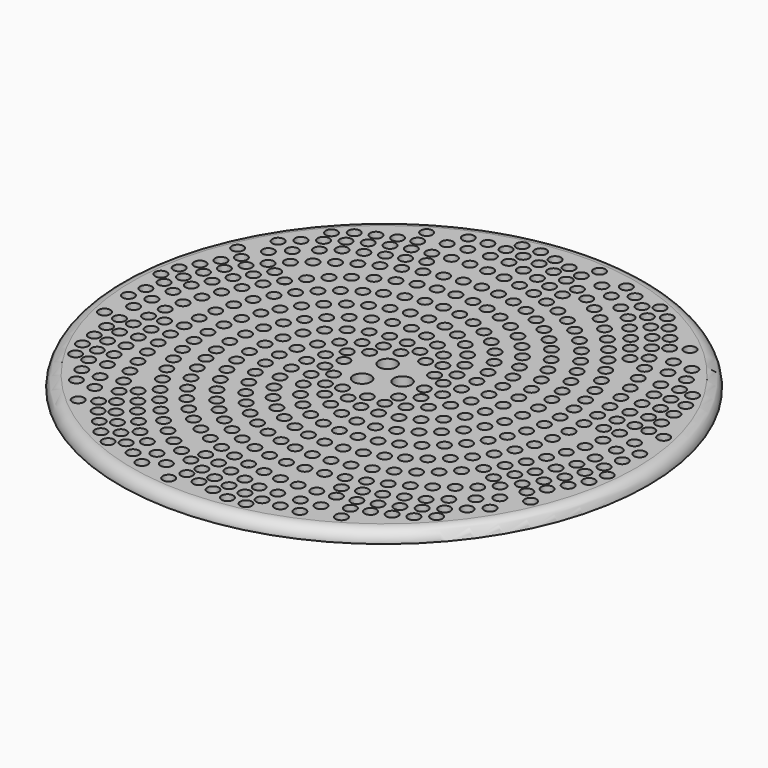
from build123d import *

# Parameters (mm, degrees)
F0_R      = 45
F1_DEPTH  = 2
F2_R      = 5.25
F3_DEPTH  = 1
F4_R      = 3.75
F5_DEPTH  = 5
F6_R      = 2
F7_R      = 1.99999
F8_R      = 1
F9_DEPTH  = 25
F10_R     = 1
F10_R_2   = 1.5
F11_DEPTH = 25


# Not quite as in the source:
# - a fillet or chamfer is up to 0.001 mm smaller than in the source, because OpenCascade refuses the exact size


with BuildPart() as f1:
    # F0 (on Top) → F1 (new body)
    with BuildSketch(Plane.XY):
        Circle(F0_R)
    extrude(amount=F1_DEPTH)

    # F2 (on face) → F3 (cut)
    with BuildSketch(Plane(origin=(0, 0, 0), x_dir=(1, 0, 0), z_dir=(0, 0, -1))):
        with Locations((0, 35)):
            Circle(F2_R)
        with Locations((-30.3108891325, -17.5)):
            Circle(F2_R)
        with Locations((30.3108891325, -17.5)):
            Circle(F2_R)
    extrude(amount=-F3_DEPTH, mode=Mode.SUBTRACT)

    # F4 (on face) → F5 (join)
    with BuildSketch(Plane(origin=(0, 0, 1), x_dir=(1, 0, 0), z_dir=(0, 0, -1))):
        with Locations((0, 35)):
            Circle(F4_R)
        with Locations((30.3108891325, -17.5)):
            Circle(F4_R)
        with Locations((-30.3108891325, -17.5)):
            Circle(F4_R)
    extrude(amount=F5_DEPTH)

    # F6
    f6_edges = [f1.edges().sort_by_distance(p)[0] for p in [
        (-34.060889, 17.5, -4),
        (-3.75, -35, -4),
        (26.560889, 17.5, -4),
    ]]
    fillet(f6_edges, radius=F6_R)

    # F7 (radius 2 in the source; OpenCascade refuses exactly that, so slightly less here)
    f7_edges = [f1.edges().sort_by_distance(p)[0] for p in [
        (-45, 0, 2),
    ]]
    fillet(f7_edges, radius=F7_R)

    # F8 (on face) → F9 (cut)
    with BuildSketch(Plane.XY.offset(2)):
        with Locations((-40.8493989427, -3.4236625268)):
            Circle(F8_R)
        with Locations((-37.2194312295, 8.0217761925)):
            Circle(F8_R)
        with Locations((-39.4834812949, 2.4710397464)):
            Circle(F8_R)
        with Locations((-38.4680309655, 5.2939567888)):
            Circle(F8_R)
        with Locations((-40.2713256638, -0.4236625268)):
            Circle(F8_R)
        with Locations((-35.7373339506, 10.6301066271)):
            Circle(F8_R)
        with Locations((-34.027593705, 13.0952208826)):
            Circle(F8_R)
        with Locations((-32.1025009246, 15.3960941487)):
            Circle(F8_R)
        with Locations((-22.7184350173, 22.804778367)):
            Circle(F8_R)
        with Locations((-27.6942880126, 19.4590303855)):
            Circle(F8_R)
        with Locations((-25.2667541466, 21.2217213197)):
            Circle(F8_R)
        with Locations((-29.981542035, 17.5177758847)):
            Circle(F8_R)
        with Locations((-20.0643504801, 24.2032901724)):
            Circle(F8_R)
        with Locations((-17.3167057976, 25.4076359278)):
            Circle(F8_R)
        with Locations((-14.4864313326, 26.4023954226)):
            Circle(F8_R)
        with Locations((-11.5849426999, 27.1648675298)):
            Circle(F8_R)
        with Locations((-8.626607772, 27.6631189269)):
            Circle(F8_R)
        with Locations((-5.6326711003, 27.8537578673)):
            Circle(F8_R)
        with Locations((5.9110662235, 25.0201439515)):
            Circle(F8_R)
        with Locations((0.3145207901, 27.1521286585)):
            Circle(F8_R)
        with Locations((3.177785049, 26.256741712)):
            Circle(F8_R)
        with Locations((-2.6372636774, 27.6878230277)):
            Circle(F8_R)
        with Locations((8.4765099907, 23.4649917798)):
            Circle(F8_R)
        with Locations((10.8377438023, 21.6144310845)):
            Circle(F8_R)
        with Locations((12.8210696775, 19.6416883073)):
            Circle(F8_R)
        with Locations((14.6696584192, 17.2789103524)):
            Circle(F8_R)
        with Locations((16.1762201169, 14.6846336033)):
            Circle(F8_R)
        with Locations((17.2872605499, 11.8979529334)):
            Circle(F8_R)
        with Locations((17.1563704418, 0.1090617956)):
            Circle(F8_R)
        with Locations((18.1599637889, 6.0055567892)):
            Circle(F8_R)
        with Locations((17.8915320419, 3.0175901902)):
            Circle(F8_R)
        with Locations((17.9579806895, 8.973891632)):
            Circle(F8_R)
        with Locations((15.9391579938, -2.6329071787)):
            Circle(F8_R)
        with Locations((14.2051991524, -5.0810466225)):
            Circle(F8_R)
        with Locations((6.3437518281, -9.104549132)):
            Circle(F8_R)
        with Locations((3.343753197, -9.1074149941)):
            Circle(F8_R)
        with Locations((9.2585771237, -8.3947650127)):
            Circle(F8_R)
        with Locations((11.9383022455, -7.0460347685)):
            Circle(F8_R)
        with Locations((0.4738705573, -8.2334735575)):
            Circle(F8_R)
        with Locations((-1.9367000752, -6.4476546346)):
            Circle(F8_R)
        with Locations((13.7998447247, 1.3167961267)):
            Circle(F8_R)
        with Locations((-9.9243185953, 23.71615921)):
            Circle(F8_R)
        with Locations((10.4837227456, -3.6369712052)):
            Circle(F8_R)
        with Locations((6.9922463043, 19.7868429251)):
            Circle(F8_R)
        with Locations((9.2535904055, 17.8154670462)):
            Circle(F8_R)
        with Locations((-25.3395240375, 15.1673810139)):
            Circle(F8_R)
        with Locations((-34.5522673419, -3.4505298548)):
            Circle(F8_R)
        with Locations((-30.4587375398, 7.7873437602)):
            Circle(F8_R)
        with Locations((4.455425912, 21.3882617638)):
            Circle(F8_R)
        with Locations((-28.9437429708, 10.3767049663)):
            Circle(F8_R)
        with Locations((-31.0354796126, -26.7804754307)):
            Circle(F8_R)
        with Locations((-34.8262341288, -15.3872795106)):
            Circle(F8_R)
        with Locations((-33.3952480854, -21.2086948657)):
            Circle(F8_R)
        with Locations((-32.3311642628, -24.0136414995)):
            Circle(F8_R)
        with Locations((13.8156903342, 10.1724943747)):
            Circle(F8_R)
        with Locations((-35.1603304054, -12.4059409391)):
            Circle(F8_R)
        with Locations((-35.2260792953, -9.4066615117)):
            Circle(F8_R)
        with Locations((-35.0210658934, -6.4136747919)):
            Circle(F8_R)
        with Locations((-31.7839124205, 5.0958921935)):
            Circle(F8_R)
        with Locations((-3.9367249114, 23.8567080462)):
            Circle(F8_R)
        with Locations((-33.8428807338, -0.5356077906)):
            Circle(F8_R)
        with Locations((-32.9150483173, 2.3173077369)):
            Circle(F8_R)
        with Locations((2.2230130322, -6.3546259156)):
            Circle(F8_R)
        with Locations((12.4246653077, -1.3494524685)):
            Circle(F8_R)
        with Locations((-27.2387077905, 12.8450758935)):
            Circle(F8_R)
        with Locations((-6.9347354779, 23.9659446861)):
            Circle(F8_R)
        with Locations((-18.4080851774, 20.8497746707)):
            Circle(F8_R)
        with Locations((14.4426337033, 7.2387353505)):
            Circle(F8_R)
        with Locations((14.4788117937, 4.2389535008)):
            Circle(F8_R)
        with Locations((12.7008584661, 12.957660421)):
            Circle(F8_R)
        with Locations((1.711714282, 22.6015409944)):
            Circle(F8_R)
        with Locations((-34.233000518, -18.3280402766)):
            Circle(F8_R)
        with Locations((8.0583573814, -5.4026446886)):
            Circle(F8_R)
        with Locations((-15.7051681295, 22.1514042001)):
            Circle(F8_R)
        with Locations((-1.172631462, 23.4264953138)):
            Circle(F8_R)
        with Locations((11.1617416099, 15.5327564005)):
            Circle(F8_R)
        with Locations((-23.239045629, 17.3093405036)):
            Circle(F8_R)
        with Locations((-12.8624434425, 23.1100054487)):
            Circle(F8_R)
        with Locations((5.2228836663, -6.3824859057)):
            Circle(F8_R)
        with Locations((-20.9289547392, 19.2233624681)):
            Circle(F8_R)
        with Locations((10.3903155584, 9.1766556577)):
            Circle(F8_R)
        with Locations((-21.9689510258, 13.3534077328)):
            Circle(F8_R)
        with Locations((10.619267903, 3.219806106)):
            Circle(F8_R)
        with Locations((-5.9735683718, 20.1178314495)):
            Circle(F8_R)
        with Locations((-2.9853568954, 19.8521395742)):
            Circle(F8_R)
        with Locations((-29.4152684516, -2.623529529)):
            Circle(F8_R)
        with Locations((-25.9252009125, -23.100850469)):
            Circle(F8_R)
        with Locations((-29.2189221137, -11.6031032863)):
            Circle(F8_R)
        with Locations((-8.967189557, 19.9223008908)):
            Circle(F8_R)
        with Locations((-29.5152540908, -8.617774601)):
            Circle(F8_R)
        with Locations((-9.3670619276, -39.908056955)):
            Circle(F8_R)
        with Locations((-19.1305992911, -32.9189174351)):
            Circle(F8_R)
        with Locations((-14.55116517, -36.7874288961)):
            Circle(F8_R)
        with Locations((-12.0415970093, -38.431225613)):
            Circle(F8_R)
        with Locations((5.1978860969, 16.350379853)):
            Circle(F8_R)
        with Locations((-21.153275701, -30.7033407289)):
            Circle(F8_R)
        with Locations((-22.9693998852, -28.3155189292)):
            Circle(F8_R)
        with Locations((-24.5627740133, -25.7736379547)):
            Circle(F8_R)
        with Locations((-28.7090155745, -14.5594515948)):
            Circle(F8_R)
        with Locations((-17.2074985133, 16.9865333939)):
            Circle(F8_R)
        with Locations((-27.0646432919, -20.3256619954)):
            Circle(F8_R)
        with Locations((-27.9909127721, -17.4722386391)):
            Circle(F8_R)
        with Locations((5.5336107188, -3.8343460826)):
            Circle(F8_R)
        with Locations((10.844953643, 6.2113050524)):
            Circle(F8_R)
        with Locations((-29.5867236821, -5.6186260389)):
            Circle(F8_R)
        with Locations((-19.6971476969, 15.3127212949)):
            Circle(F8_R)
        with Locations((-27.1476438075, 6.0478210472)):
            Circle(F8_R)
        with Locations((7.4295142253, 14.3454270114)):
            Circle(F8_R)
        with Locations((9.2220104465, 11.9398174636)):
            Circle(F8_R)
        with Locations((2.6588886425, 17.9483447858)):
            Circle(F8_R)
        with Locations((-11.900046532, 19.2911511746)):
            Circle(F8_R)
        with Locations((-16.9221274095, -34.9493489036)):
            Circle(F8_R)
        with Locations((9.6949429396, 0.3657522589)):
            Circle(F8_R)
        with Locations((-25.7260166227, 8.6895962359)):
            Circle(F8_R)
        with Locations((-14.7184272393, 18.2631773478)):
            Circle(F8_R)
        with Locations((-0.0998864904, 19.1269710057)):
            Circle(F8_R)
        with Locations((-28.9749579218, 0.3439823307)):
            Circle(F8_R)
        with Locations((-23.9896557173, 11.1360325842)):
            Circle(F8_R)
        with Locations((7.976932734, -2.0936055706)):
            Circle(F8_R)
        with Locations((-28.2310890167, 3.2502959841)):
            Circle(F8_R)
        with Locations((3.0120390027, 13.5313446305)):
            Circle(F8_R)
        with Locations((-25.6221908617, -2.1098916326)):
            Circle(F8_R)
        with Locations((6.698613657, 8.8467269218)):
            Circle(F8_R)
        with Locations((-16.6576829639, 12.7644921402)):
            Circle(F8_R)
        with Locations((-14.0839993308, 14.3059695343)):
            Circle(F8_R)
        with Locations((-22.2553801054, -19.4123409623)):
            Circle(F8_R)
        with Locations((-7.3955888997, -33.927431373)):
            Circle(F8_R)
        with Locations((-16.8184715547, -26.5615592524)):
            Circle(F8_R)
        with Locations((-18.9646433987, 10.8466982116)):
            Circle(F8_R)
        with Locations((-18.8129413347, -24.3205571782)):
            Circle(F8_R)
        with Locations((15.879255039, -37.7921171474)):
            Circle(F8_R)
        with Locations((3.8722742507, -37.8766477722)):
            Circle(F8_R)
        with Locations((9.8509682644, -38.3146154469)):
            Circle(F8_R)
        with Locations((12.847451023, -38.1693877717)):
            Circle(F8_R)
        with Locations((-5.4053339597, 16.2829759564)):
            Circle(F8_R)
        with Locations((0.9336113478, -37.2731079285)):
            Circle(F8_R)
        with Locations((-1.9391904202, -36.4088105248)):
            Circle(F8_R)
        with Locations((-4.722337318, -35.2889474326)):
            Circle(F8_R)
        with Locations((-14.6682505627, -28.6535797316)):
            Circle(F8_R)
        with Locations((-23.9055925445, 3.6280803362)):
            Circle(F8_R)
        with Locations((-9.9486320059, -32.3520041617)):
            Circle(F8_R)
        with Locations((-12.3751999241, -30.5879837145)):
            Circle(F8_R)
        with Locations((6.7305571913, 0.1505236293)):
            Circle(F8_R)
        with Locations((5.1228382931, 11.3995551578)):
            Circle(F8_R)
        with Locations((-20.6336167429, -21.9362037945)):
            Circle(F8_R)
        with Locations((-24.9359189771, 0.8105588293)):
            Circle(F8_R)
        with Locations((-25.5177252176, -11.0641946584)):
            Circle(F8_R)
        with Locations((-2.421427167, 15.9726531371)):
            Circle(F8_R)
        with Locations((0.4427145534, 15.0800769747)):
            Circle(F8_R)
        with Locations((-8.3986862702, 16.0833714841)):
            Circle(F8_R)
        with Locations((-20.9663940384, 8.6121972882)):
            Circle(F8_R)
        with Locations((6.8524232075, -38.2211941341)):
            Circle(F8_R)
        with Locations((7.6283898139, 5.9944442749)):
            Circle(F8_R)
        with Locations((-25.9204011611, -8.091342142)):
            Circle(F8_R)
        with Locations((-22.6422840721, 6.1239463775)):
            Circle(F8_R)
        with Locations((-11.3233613464, 15.4153327886)):
            Circle(F8_R)
        with Locations((-23.6434211111, -16.7527654009)):
            Circle(F8_R)
        with Locations((-25.9536348865, -5.0915262277)):
            Circle(F8_R)
        with Locations((7.6840646233, 2.9949609334)):
            Circle(F8_R)
        with Locations((-24.7499068293, -13.9642730923)):
            Circle(F8_R)
        with Locations((-5.5167340766, 12.717519868)):
            Circle(F8_R)
        with Locations((-19.4886246546, -16.767284107)):
            Circle(F8_R)
        with Locations((0.2193166715, 11.0944987427)):
            Circle(F8_R)
        with Locations((-20.9791288377, 0.5355506824)):
            Circle(F8_R)
        with Locations((-19.8030327194, 3.2954053743)):
            Circle(F8_R)
        with Locations((-6.5946929914, -28.7862979492)):
            Circle(F8_R)
        with Locations((13.9588867059, -31.7948866435)):
            Circle(F8_R)
        with Locations((2.0060634993, -31.3744023783)):
            Circle(F8_R)
        with Locations((-21.7182480467, -2.3719745187)):
            Circle(F8_R)
        with Locations((-0.9247244171, -30.7337135386)):
            Circle(F8_R)
        with Locations((35.0602362968, -21.2408730963)):
            Circle(F8_R)
        with Locations((25.3960706425, -28.3667860402)):
            Circle(F8_R)
        with Locations((30.4903666439, -25.2069211629)):
            Circle(F8_R)
        with Locations((32.8292094332, -23.3281411313)):
            Circle(F8_R)
        with Locations((-13.9439001643, 9.9960286825)):
            Circle(F8_R)
        with Locations((22.663890594, -29.6058147657)):
            Circle(F8_R)
        with Locations((19.8317238747, -30.5951739899)):
            Circle(F8_R)
        with Locations((16.9218717264, -31.3250784185)):
            Circle(F8_R)
        with Locations((4.9752876087, -31.8030143102)):
            Circle(F8_R)
        with Locations((-21.4725627448, -11.116176096)):
            Circle(F8_R)
        with Locations((10.9674185648, -32.0209803425)):
            Circle(F8_R)
        with Locations((7.9674186773, -32.0201586583)):
            Circle(F8_R)
        with Locations((5.35665958, 4.0778984309)):
            Circle(F8_R)
        with Locations((-2.5560271659, 12.2335626496)):
            Circle(F8_R)
        with Locations((-3.7991695187, -29.8748972847)):
            Circle(F8_R)
        with Locations((-20.6500167488, -14.0012095593)):
            Circle(F8_R)
        with Locations((-14.1409029101, -23.9500640627)):
            Circle(F8_R)
        with Locations((-11.3474656827, 11.4988686549)):
            Circle(F8_R)
        with Locations((-8.5056832518, 12.4602596345)):
            Circle(F8_R)
        with Locations((-16.2482484885, 8.0750969292)):
            Circle(F8_R)
        with Locations((-22.0242916437, -5.3563232444)):
            Circle(F8_R)
        with Locations((28.0095810645, -26.8938422959)):
            Circle(F8_R)
        with Locations((2.6480510587, 9.3334623216)):
            Circle(F8_R)
        with Locations((-16.2140734581, -21.7816628362)):
            Circle(F8_R)
        with Locations((-21.9175579723, -8.3544239638)):
            Circle(F8_R)
        with Locations((-18.221697035, 5.8155613941)):
            Circle(F8_R)
        with Locations((-9.2809010463, -27.450526155)):
            Circle(F8_R)
        with Locations((-18.0042076607, -19.3742950752)):
            Circle(F8_R)
        with Locations((4.4561449982, 6.9395541559)):
            Circle(F8_R)
        with Locations((-11.8151014515, -25.8449644756)):
            Circle(F8_R)
        with Locations((-11.9383022455, 7.0460347685)):
            Circle(F8_R)
        with Locations((-5.9110662235, -25.0201439515)):
            Circle(F8_R)
        with Locations((-6.3437518281, 9.104549132)):
            Circle(F8_R)
        with Locations((-17.2872605499, -11.8979529334)):
            Circle(F8_R)
        with Locations((-17.9579806895, -8.973891632)):
            Circle(F8_R)
        with Locations((11.5849426999, -27.1648675298)):
            Circle(F8_R)
        with Locations((29.981542035, -17.5177758847)):
            Circle(F8_R)
        with Locations((20.0643504801, -24.2032901724)):
            Circle(F8_R)
        with Locations((-16.1762201169, -14.6846336033)):
            Circle(F8_R)
        with Locations((17.3167057976, -25.4076359278)):
            Circle(F8_R)
        with Locations((40.8493989427, 3.4236625268)):
            Circle(F8_R)
        with Locations((37.2194312295, -8.0217761925)):
            Circle(F8_R)
        with Locations((39.4834812949, -2.4710397464)):
            Circle(F8_R)
        with Locations((40.2713256638, 0.4236625268)):
            Circle(F8_R)
        with Locations((-17.1563704418, -0.1090617956)):
            Circle(F8_R)
        with Locations((35.7373339506, -10.6301066271)):
            Circle(F8_R)
        with Locations((34.027593705, -13.0952208826)):
            Circle(F8_R)
        with Locations((32.1025009246, -15.3960941487)):
            Circle(F8_R)
        with Locations((22.7184350173, -22.804778367)):
            Circle(F8_R)
        with Locations((-10.8377438023, -21.6144310845)):
            Circle(F8_R)
        with Locations((27.6942880126, -19.4590303855)):
            Circle(F8_R)
        with Locations((25.2667541466, -21.2217213197)):
            Circle(F8_R)
        with Locations((1.9367000752, 6.4476546346)):
            Circle(F8_R)
        with Locations((-9.2585771237, 8.3947650127)):
            Circle(F8_R)
        with Locations((14.4864313326, -26.4023954226)):
            Circle(F8_R)
        with Locations((-8.4765099907, -23.4649917798)):
            Circle(F8_R)
        with Locations((2.6372636774, -27.6878230277)):
            Circle(F8_R)
        with Locations((-15.9391579938, 2.6329071787)):
            Circle(F8_R)
        with Locations((-14.2051991524, 5.0810466225)):
            Circle(F8_R)
        with Locations((-17.8915320419, -3.0175901902)):
            Circle(F8_R)
        with Locations((-14.6696584192, -17.2789103524)):
            Circle(F8_R)
        with Locations((38.4680309655, -5.2939567888)):
            Circle(F8_R)
        with Locations((-3.343753197, 9.1074149941)):
            Circle(F8_R)
        with Locations((-0.3145207901, -27.1521286585)):
            Circle(F8_R)
        with Locations((-12.8210696775, -19.6416883073)):
            Circle(F8_R)
        with Locations((-18.1599637889, -6.0055567892)):
            Circle(F8_R)
        with Locations((8.626607772, -27.6631189269)):
            Circle(F8_R)
        with Locations((-3.177785049, -26.256741712)):
            Circle(F8_R)
        with Locations((-0.4738705573, 8.2334735575)):
            Circle(F8_R)
        with Locations((5.6326711003, -27.8537578673)):
            Circle(F8_R)
        with Locations((-13.7998447247, -1.3167961267)):
            Circle(F8_R)
        with Locations((9.9243185953, -23.71615921)):
            Circle(F8_R)
        with Locations((-10.4837227456, 3.6369712052)):
            Circle(F8_R)
        with Locations((-6.9922463043, -19.7868429251)):
            Circle(F8_R)
        with Locations((-9.2535904055, -17.8154670462)):
            Circle(F8_R)
        with Locations((25.3395240375, -15.1673810139)):
            Circle(F8_R)
        with Locations((34.5522673419, 3.4505298548)):
            Circle(F8_R)
        with Locations((30.4587375398, -7.7873437602)):
            Circle(F8_R)
        with Locations((-4.455425912, -21.3882617638)):
            Circle(F8_R)
        with Locations((28.9437429708, -10.3767049663)):
            Circle(F8_R)
        with Locations((31.0354796126, 26.7804754307)):
            Circle(F8_R)
        with Locations((34.8262341288, 15.3872795106)):
            Circle(F8_R)
        with Locations((33.3952480854, 21.2086948657)):
            Circle(F8_R)
        with Locations((32.3311642628, 24.0136414995)):
            Circle(F8_R)
        with Locations((-13.8156903342, -10.1724943747)):
            Circle(F8_R)
        with Locations((35.1603304054, 12.4059409391)):
            Circle(F8_R)
        with Locations((35.2260792953, 9.4066615117)):
            Circle(F8_R)
        with Locations((35.0210658934, 6.4136747919)):
            Circle(F8_R)
        with Locations((31.7839124205, -5.0958921935)):
            Circle(F8_R)
        with Locations((3.9367249114, -23.8567080462)):
            Circle(F8_R)
        with Locations((33.8428807338, 0.5356077906)):
            Circle(F8_R)
        with Locations((32.9150483173, -2.3173077369)):
            Circle(F8_R)
        with Locations((-2.2230130322, 6.3546259156)):
            Circle(F8_R)
        with Locations((-12.4246653077, 1.3494524685)):
            Circle(F8_R)
        with Locations((27.2387077905, -12.8450758935)):
            Circle(F8_R)
        with Locations((6.9347354779, -23.9659446861)):
            Circle(F8_R)
        with Locations((18.4080851774, -20.8497746707)):
            Circle(F8_R)
        with Locations((-14.4426337033, -7.2387353505)):
            Circle(F8_R)
        with Locations((-14.4788117937, -4.2389535008)):
            Circle(F8_R)
        with Locations((-12.7008584661, -12.957660421)):
            Circle(F8_R)
        with Locations((-1.711714282, -22.6015409944)):
            Circle(F8_R)
        with Locations((34.233000518, 18.3280402766)):
            Circle(F8_R)
        with Locations((-8.0583573814, 5.4026446886)):
            Circle(F8_R)
        with Locations((15.7051681295, -22.1514042001)):
            Circle(F8_R)
        with Locations((1.172631462, -23.4264953138)):
            Circle(F8_R)
        with Locations((-11.1617416099, -15.5327564005)):
            Circle(F8_R)
        with Locations((23.239045629, -17.3093405036)):
            Circle(F8_R)
        with Locations((12.8624434425, -23.1100054487)):
            Circle(F8_R)
        with Locations((-5.2228836663, 6.3824859057)):
            Circle(F8_R)
        with Locations((20.9289547392, -19.2233624681)):
            Circle(F8_R)
        with Locations((-10.3903155584, -9.1766556577)):
            Circle(F8_R)
        with Locations((21.9689510258, -13.3534077328)):
            Circle(F8_R)
        with Locations((-10.619267903, -3.219806106)):
            Circle(F8_R)
        with Locations((5.9735683718, -20.1178314495)):
            Circle(F8_R)
        with Locations((2.9853568954, -19.8521395742)):
            Circle(F8_R)
        with Locations((29.4152684516, 2.623529529)):
            Circle(F8_R)
        with Locations((25.9252009125, 23.100850469)):
            Circle(F8_R)
        with Locations((29.2189221137, 11.6031032863)):
            Circle(F8_R)
        with Locations((8.967189557, -19.9223008908)):
            Circle(F8_R)
        with Locations((29.5152540908, 8.617774601)):
            Circle(F8_R)
        with Locations((9.3670619276, 39.908056955)):
            Circle(F8_R)
        with Locations((19.1305992911, 32.9189174351)):
            Circle(F8_R)
        with Locations((14.55116517, 36.7874288961)):
            Circle(F8_R)
        with Locations((12.0415970093, 38.431225613)):
            Circle(F8_R)
        with Locations((-5.1978860969, -16.350379853)):
            Circle(F8_R)
        with Locations((21.153275701, 30.7033407289)):
            Circle(F8_R)
        with Locations((22.9693998852, 28.3155189292)):
            Circle(F8_R)
        with Locations((24.5627740133, 25.7736379547)):
            Circle(F8_R)
        with Locations((28.7090155745, 14.5594515948)):
            Circle(F8_R)
        with Locations((17.2074985133, -16.9865333939)):
            Circle(F8_R)
        with Locations((27.0646432919, 20.3256619954)):
            Circle(F8_R)
        with Locations((27.9909127721, 17.4722386391)):
            Circle(F8_R)
        with Locations((-5.5336107188, 3.8343460826)):
            Circle(F8_R)
        with Locations((-10.844953643, -6.2113050524)):
            Circle(F8_R)
        with Locations((29.5867236821, 5.6186260389)):
            Circle(F8_R)
        with Locations((19.6971476969, -15.3127212949)):
            Circle(F8_R)
        with Locations((27.1476438075, -6.0478210472)):
            Circle(F8_R)
        with Locations((-7.4295142253, -14.3454270114)):
            Circle(F8_R)
        with Locations((-9.2220104465, -11.9398174636)):
            Circle(F8_R)
        with Locations((-2.6588886425, -17.9483447858)):
            Circle(F8_R)
        with Locations((11.900046532, -19.2911511746)):
            Circle(F8_R)
        with Locations((16.9221274095, 34.9493489036)):
            Circle(F8_R)
        with Locations((-9.6949429396, -0.3657522589)):
            Circle(F8_R)
        with Locations((25.7260166227, -8.6895962359)):
            Circle(F8_R)
        with Locations((14.7184272393, -18.2631773478)):
            Circle(F8_R)
        with Locations((0.0998864904, -19.1269710057)):
            Circle(F8_R)
        with Locations((28.9749579218, -0.3439823307)):
            Circle(F8_R)
        with Locations((23.9896557173, -11.1360325842)):
            Circle(F8_R)
        with Locations((-7.976932734, 2.0936055706)):
            Circle(F8_R)
        with Locations((28.2310890167, -3.2502959841)):
            Circle(F8_R)
        with Locations((-3.0120390027, -13.5313446305)):
            Circle(F8_R)
        with Locations((25.6221908617, 2.1098916326)):
            Circle(F8_R)
        with Locations((-6.698613657, -8.8467269218)):
            Circle(F8_R)
        with Locations((16.6576829639, -12.7644921402)):
            Circle(F8_R)
        with Locations((14.0839993308, -14.3059695343)):
            Circle(F8_R)
        with Locations((22.2553801054, 19.4123409623)):
            Circle(F8_R)
        with Locations((7.3955888997, 33.927431373)):
            Circle(F8_R)
        with Locations((16.8184715547, 26.5615592524)):
            Circle(F8_R)
        with Locations((18.9646433987, -10.8466982116)):
            Circle(F8_R)
        with Locations((18.8129413347, 24.3205571782)):
            Circle(F8_R)
        with Locations((-15.879255039, 37.7921171474)):
            Circle(F8_R)
        with Locations((-3.8722742507, 37.8766477722)):
            Circle(F8_R)
        with Locations((-9.8509682644, 38.3146154469)):
            Circle(F8_R)
        with Locations((-12.847451023, 38.1693877717)):
            Circle(F8_R)
        with Locations((5.4053339597, -16.2829759564)):
            Circle(F8_R)
        with Locations((-0.9336113478, 37.2731079285)):
            Circle(F8_R)
        with Locations((1.9391904202, 36.4088105248)):
            Circle(F8_R)
        with Locations((4.722337318, 35.2889474326)):
            Circle(F8_R)
        with Locations((14.6682505627, 28.6535797316)):
            Circle(F8_R)
        with Locations((23.9055925445, -3.6280803362)):
            Circle(F8_R)
        with Locations((9.9486320059, 32.3520041617)):
            Circle(F8_R)
        with Locations((12.3751999241, 30.5879837145)):
            Circle(F8_R)
        with Locations((-6.7305571913, -0.1505236293)):
            Circle(F8_R)
        with Locations((-5.1228382931, -11.3995551578)):
            Circle(F8_R)
        with Locations((20.6336167429, 21.9362037945)):
            Circle(F8_R)
        with Locations((24.9359189771, -0.8105588293)):
            Circle(F8_R)
        with Locations((25.5177252176, 11.0641946584)):
            Circle(F8_R)
        with Locations((2.421427167, -15.9726531371)):
            Circle(F8_R)
        with Locations((-0.4427145534, -15.0800769747)):
            Circle(F8_R)
        with Locations((8.3986862702, -16.0833714841)):
            Circle(F8_R)
        with Locations((20.9663940384, -8.6121972882)):
            Circle(F8_R)
        with Locations((-6.8524232075, 38.2211941341)):
            Circle(F8_R)
        with Locations((-7.6283898139, -5.9944442749)):
            Circle(F8_R)
        with Locations((25.9204011611, 8.091342142)):
            Circle(F8_R)
        with Locations((22.6422840721, -6.1239463775)):
            Circle(F8_R)
        with Locations((11.3233613464, -15.4153327886)):
            Circle(F8_R)
        with Locations((23.6434211111, 16.7527654009)):
            Circle(F8_R)
        with Locations((25.9536348865, 5.0915262277)):
            Circle(F8_R)
        with Locations((-7.6840646233, -2.9949609334)):
            Circle(F8_R)
        with Locations((24.7499068293, 13.9642730923)):
            Circle(F8_R)
        with Locations((5.5167340766, -12.717519868)):
            Circle(F8_R)
        with Locations((19.4886246546, 16.767284107)):
            Circle(F8_R)
        with Locations((-0.2193166715, -11.0944987427)):
            Circle(F8_R)
        with Locations((20.9791288377, -0.5355506824)):
            Circle(F8_R)
        with Locations((19.8030327194, -3.2954053743)):
            Circle(F8_R)
        with Locations((6.5946929914, 28.7862979492)):
            Circle(F8_R)
        with Locations((-13.9588867059, 31.7948866435)):
            Circle(F8_R)
        with Locations((-2.0060634993, 31.3744023783)):
            Circle(F8_R)
        with Locations((21.7182480467, 2.3719745187)):
            Circle(F8_R)
        with Locations((0.9247244171, 30.7337135386)):
            Circle(F8_R)
        with Locations((-35.0602362968, 21.2408730963)):
            Circle(F8_R)
        with Locations((-25.3960706425, 28.3667860402)):
            Circle(F8_R)
        with Locations((-30.4903666439, 25.2069211629)):
            Circle(F8_R)
        with Locations((-32.8292094332, 23.3281411313)):
            Circle(F8_R)
        with Locations((13.9439001643, -9.9960286825)):
            Circle(F8_R)
        with Locations((-22.663890594, 29.6058147657)):
            Circle(F8_R)
        with Locations((-19.8317238747, 30.5951739899)):
            Circle(F8_R)
        with Locations((-16.9218717264, 31.3250784185)):
            Circle(F8_R)
        with Locations((-4.9752876087, 31.8030143102)):
            Circle(F8_R)
        with Locations((21.4725627448, 11.116176096)):
            Circle(F8_R)
        with Locations((-10.9674185648, 32.0209803425)):
            Circle(F8_R)
        with Locations((-7.9674186773, 32.0201586583)):
            Circle(F8_R)
        with Locations((-5.35665958, -4.0778984309)):
            Circle(F8_R)
        with Locations((2.5560271659, -12.2335626496)):
            Circle(F8_R)
        with Locations((3.7991695187, 29.8748972847)):
            Circle(F8_R)
        with Locations((20.6500167488, 14.0012095593)):
            Circle(F8_R)
        with Locations((14.1409029101, 23.9500640627)):
            Circle(F8_R)
        with Locations((11.3474656827, -11.4988686549)):
            Circle(F8_R)
        with Locations((8.5056832518, -12.4602596345)):
            Circle(F8_R)
        with Locations((16.2482484885, -8.0750969292)):
            Circle(F8_R)
        with Locations((22.0242916437, 5.3563232444)):
            Circle(F8_R)
        with Locations((-28.0095810645, 26.8938422959)):
            Circle(F8_R)
        with Locations((-2.6480510587, -9.3334623216)):
            Circle(F8_R)
        with Locations((16.2140734581, 21.7816628362)):
            Circle(F8_R)
        with Locations((21.9175579723, 8.3544239638)):
            Circle(F8_R)
        with Locations((18.221697035, -5.8155613941)):
            Circle(F8_R)
        with Locations((9.2809010463, 27.450526155)):
            Circle(F8_R)
        with Locations((18.0042076607, 19.3742950752)):
            Circle(F8_R)
        with Locations((-4.4561449982, -6.9395541559)):
            Circle(F8_R)
        with Locations((11.8151014515, 25.8449644756)):
            Circle(F8_R)
    extrude(amount=-F9_DEPTH, mode=Mode.SUBTRACT)

    # F10 (on face) → F11 (cut)
    with BuildSketch(Plane.XY.offset(2)):
        with Locations((38.0169600248, -16.3124445826)):
            Circle(F10_R)
        with Locations((35.9479473242, -14.5082109163)):
            Circle(F10_R)
        with Locations((31.5856789797, -11.6352651169)):
            Circle(F10_R)
        with Locations((29.9237966537, -14.094513841)):
            Circle(F10_R)
        with Locations((37.5461820224, -12.1688387011)):
            Circle(F10_R)
        with Locations((33.1839136779, -9.2958929017)):
            Circle(F10_R)
        with Locations((39.0696208635, -9.6030315038)):
            Circle(F10_R)
        with Locations((34.707352519, -6.7300857045)):
            Circle(F10_R)
        with Locations((40.528966085, -6.9981851269)):
            Circle(F10_R)
        with Locations((36.1666977406, -4.1252393275)):
            Circle(F10_R)
        with Locations((41.2958357194, -4.0729459728)):
            Circle(F10_R)
        with Locations((36.9335673749, -1.2000001734)):
            Circle(F10_R)
        with Locations((37.7309508622, 2.3215697147)):
            Circle(F10_R)
        with Locations((38.3053118558, 5.4717249956)):
            Circle(F10_R)
        with Locations((29.160396021, 24.0558858246)):
            Circle(F10_R)
        with Locations((27.7734490091, 26.9420159032)):
            Circle(F10_R)
        with Locations((32.4934074031, 6.1860651409)):
            Circle(F10_R)
        with Locations((37.5281632561, 12.2242947617)):
            Circle(F10_R)
        with Locations((32.3103388598, 11.9844797379)):
            Circle(F10_R)
        with Locations((37.2525075376, 15.1955312721)):
            Circle(F10_R)
        with Locations((32.0346831414, 14.9557162483)):
            Circle(F10_R)
        with Locations((36.9020523377, 18.160677858)):
            Circle(F10_R)
        with Locations((31.6842279414, 17.9208628342)):
            Circle(F10_R)
        with Locations((37.6102127119, 9.3922840981)):
            Circle(F10_R)
        with Locations((35.8030504701, 20.9780007078)):
            Circle(F10_R)
        with Locations((40.344581089, 9.1487635525)):
            Circle(F10_R)
        with Locations((30.5852260739, 20.738185684)):
            Circle(F10_R)
        with Locations((32.3923883157, 9.1524690743)):
            Circle(F10_R)
        with Locations((9.4515610251, 36.6016711789)):
            Circle(F10_R)
        with Locations((6.6330726258, 38.1213724613)):
            Circle(F10_R)
        with Locations((22.6516409347, 24.1037774955)):
            Circle(F10_R)
        with Locations((23.1756616612, 31.948163114)):
            Circle(F10_R)
        with Locations((19.0953127853, 28.6871884551)):
            Circle(F10_R)
        with Locations((21.2062024985, 34.1899175792)):
            Circle(F10_R)
        with Locations((17.1258536226, 30.9289429203)):
            Circle(F10_R)
        with Locations((19.1798088519, 36.3827791599)):
            Circle(F10_R)
        with Locations((15.099459976, 33.121804501)):
            Circle(F10_R)
        with Locations((24.9066551678, 29.705245819)):
            Circle(F10_R)
        with Locations((16.6347168422, 38.0160641341)):
            Circle(F10_R)
        with Locations((27.2619434391, 31.1154549655)):
            Circle(F10_R)
        with Locations((12.5543679662, 34.7550894751)):
            Circle(F10_R)
        with Locations((20.8263062919, 26.4442711601)):
            Circle(F10_R)
        with Locations((-13.8674490355, 35.166862188)):
            Circle(F10_R)
        with Locations((-17.0409120507, 34.739660437)):
            Circle(F10_R)
        with Locations((4.1577175302, 32.8146661042)):
            Circle(F10_R)
        with Locations((-0.0291549764, 39.4689190349)):
            Circle(F10_R)
        with Locations((-1.4134737474, 34.4323662241)):
            Circle(F10_R)
        with Locations((-2.9401511227, 40.1249174436)):
            Circle(F10_R)
        with Locations((-4.3244698937, 35.0883646329)):
            Circle(F10_R)
        with Locations((-5.8684697175, 40.7078954279)):
            Circle(F10_R)
        with Locations((-7.2527884885, 35.6713426171)):
            Circle(F10_R)
        with Locations((2.6896018956, 38.6718132812)):
            Circle(F10_R)
        with Locations((-8.8875132263, 40.5332831796)):
            Circle(F10_R)
        with Locations((3.7661699948, 41.1971001572)):
            Circle(F10_R)
        with Locations((-10.2718319973, 35.4967303688)):
            Circle(F10_R)
        with Locations((1.3052831247, 33.6352604704)):
            Circle(F10_R)
        with Locations((-31.8895649019, 20.2995071189)):
            Circle(F10_R)
        with Locations((-34.2058475231, 18.0885788833)):
            Circle(F10_R)
        with Locations((-15.9243126551, 28.9914675905)):
            Circle(F10_R)
        with Locations((-23.222835404, 31.9138893837)):
            Circle(F10_R)
        with Locations((-21.3823613508, 27.0255504086)):
            Circle(F10_R)
        with Locations((-25.9634669471, 30.7335626404)):
            Circle(F10_R)
        with Locations((-24.1229928939, 25.8452236653)):
            Circle(F10_R)
        with Locations((-28.6751923168, 29.4839792529)):
            Circle(F10_R)
        with Locations((-26.8347182636, 24.5956402779)):
            Circle(F10_R)
        with Locations((-20.5547878844, 32.8670624766)):
            Circle(F10_R)
        with Locations((-31.0150153178, 27.5681657261)):
            Circle(F10_R)
        with Locations((-21.1681523801, 35.5428533267)):
            Circle(F10_R)
        with Locations((-29.1745412645, 22.6798267511)):
            Circle(F10_R)
        with Locations((-18.7143138312, 27.9787235015)):
            Circle(F10_R)
        with Locations((-37.7309508622, -2.3215697147)):
            Circle(F10_R)
        with Locations((-38.3053118558, -5.4717249956)):
            Circle(F10_R)
        with Locations((-29.9237966537, 14.094513841)):
            Circle(F10_R)
        with Locations((-37.5461820224, 12.1688387011)):
            Circle(F10_R)
        with Locations((-33.1839136779, 9.2958929017)):
            Circle(F10_R)
        with Locations((-39.0696208635, 9.6030315038)):
            Circle(F10_R)
        with Locations((-34.707352519, 6.7300857045)):
            Circle(F10_R)
        with Locations((-40.528966085, 6.9981851269)):
            Circle(F10_R)
        with Locations((-36.1666977406, 4.1252393275)):
            Circle(F10_R)
        with Locations((-35.9479473242, 14.5082109163)):
            Circle(F10_R)
        with Locations((-41.2958357194, 4.0729459728)):
            Circle(F10_R)
        with Locations((-38.0169600248, 16.3124445826)):
            Circle(F10_R)
        with Locations((-36.9335673749, 1.2000001734)):
            Circle(F10_R)
        with Locations((-31.5856789797, 11.6352651169)):
            Circle(F10_R)
        with Locations((-29.160396021, -24.0558858246)):
            Circle(F10_R)
        with Locations((-27.7734490091, -26.9420159032)):
            Circle(F10_R)
        with Locations((-32.4934074031, -6.1860651409)):
            Circle(F10_R)
        with Locations((-37.5281632561, -12.2242947617)):
            Circle(F10_R)
        with Locations((-32.3103388598, -11.9844797379)):
            Circle(F10_R)
        with Locations((-37.2525075376, -15.1955312721)):
            Circle(F10_R)
        with Locations((-32.0346831414, -14.9557162483)):
            Circle(F10_R)
        with Locations((-36.9020523377, -18.160677858)):
            Circle(F10_R)
        with Locations((-31.6842279414, -17.9208628342)):
            Circle(F10_R)
        with Locations((-37.6102127119, -9.3922840981)):
            Circle(F10_R)
        with Locations((-35.8030504701, -20.9780007078)):
            Circle(F10_R)
        with Locations((-40.344581089, -9.1487635525)):
            Circle(F10_R)
        with Locations((-30.5852260739, -20.738185684)):
            Circle(F10_R)
        with Locations((-32.3923883157, -9.1524690743)):
            Circle(F10_R)
        with Locations((-9.4515610251, -36.6016711789)):
            Circle(F10_R)
        with Locations((-6.6330726258, -38.1213724613)):
            Circle(F10_R)
        with Locations((-22.6516409347, -24.1037774955)):
            Circle(F10_R)
        with Locations((-23.1756616612, -31.948163114)):
            Circle(F10_R)
        with Locations((-19.0953127853, -28.6871884551)):
            Circle(F10_R)
        with Locations((-21.2062024985, -34.1899175792)):
            Circle(F10_R)
        with Locations((-17.1258536226, -30.9289429203)):
            Circle(F10_R)
        with Locations((-19.1798088519, -36.3827791599)):
            Circle(F10_R)
        with Locations((-15.099459976, -33.121804501)):
            Circle(F10_R)
        with Locations((-24.9066551678, -29.705245819)):
            Circle(F10_R)
        with Locations((-16.6347168422, -38.0160641341)):
            Circle(F10_R)
        with Locations((-27.2619434391, -31.1154549655)):
            Circle(F10_R)
        with Locations((-12.5543679662, -34.7550894751)):
            Circle(F10_R)
        with Locations((-20.8263062919, -26.4442711601)):
            Circle(F10_R)
        with Locations((13.8674490355, -35.166862188)):
            Circle(F10_R)
        with Locations((17.0409120507, -34.739660437)):
            Circle(F10_R)
        with Locations((-4.1577175302, -32.8146661042)):
            Circle(F10_R)
        with Locations((0.0291549764, -39.4689190349)):
            Circle(F10_R)
        with Locations((1.4134737474, -34.4323662241)):
            Circle(F10_R)
        with Locations((2.9401511227, -40.1249174436)):
            Circle(F10_R)
        with Locations((4.3244698937, -35.0883646329)):
            Circle(F10_R)
        with Locations((5.8684697175, -40.7078954279)):
            Circle(F10_R)
        with Locations((7.2527884885, -35.6713426171)):
            Circle(F10_R)
        with Locations((-2.6896018956, -38.6718132812)):
            Circle(F10_R)
        with Locations((8.8875132263, -40.5332831796)):
            Circle(F10_R)
        with Locations((-3.7661699948, -41.1971001572)):
            Circle(F10_R)
        with Locations((10.2718319973, -35.4967303688)):
            Circle(F10_R)
        with Locations((-1.3052831247, -33.6352604704)):
            Circle(F10_R)
        with Locations((31.8895649019, -20.2995071189)):
            Circle(F10_R)
        with Locations((34.2058475231, -18.0885788833)):
            Circle(F10_R)
        with Locations((15.9243126551, -28.9914675905)):
            Circle(F10_R)
        with Locations((23.222835404, -31.9138893837)):
            Circle(F10_R)
        with Locations((21.3823613508, -27.0255504086)):
            Circle(F10_R)
        with Locations((25.9634669471, -30.7335626404)):
            Circle(F10_R)
        with Locations((24.1229928939, -25.8452236653)):
            Circle(F10_R)
        with Locations((28.6751923168, -29.4839792529)):
            Circle(F10_R)
        with Locations((26.8347182636, -24.5956402779)):
            Circle(F10_R)
        with Locations((20.5547878844, -32.8670624766)):
            Circle(F10_R)
        with Locations((31.0150153178, -27.5681657261)):
            Circle(F10_R)
        with Locations((21.1681523801, -35.5428533267)):
            Circle(F10_R)
        with Locations((29.1745412645, -22.6798267511)):
            Circle(F10_R)
        with Locations((18.7143138312, -27.9787235015)):
            Circle(F10_R)
        with Locations((3.1448563095, 0)):
            Circle(F10_R_2)
        with Locations((-1.5724281548, 2.7235254553)):
            Circle(F10_R_2)
        with Locations((-1.5724281548, -2.7235254553)):
            Circle(F10_R_2)
    extrude(amount=-F11_DEPTH, mode=Mode.SUBTRACT)


solid = f1.part
